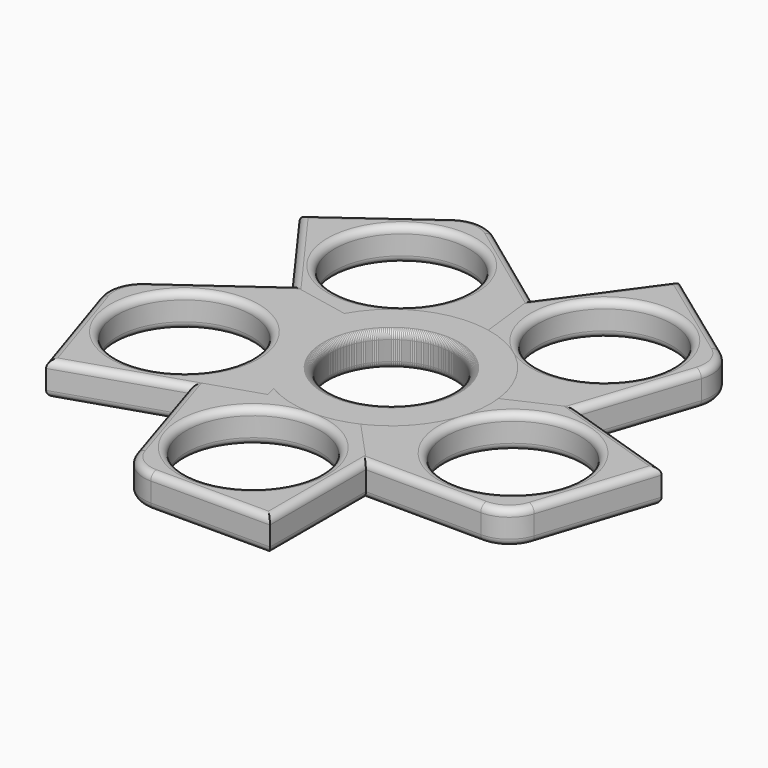
from build123d import *

# Parameters (mm, degrees)
F0_R     = 18.95
F0_R_2   = 10.95
F1_DEPTH = 6
F2_R     = 12.025
F3_DEPTH = 6
F4_R     = 1.27
F5_R     = 1.27
F6_COUNT = 5


# Not quite as in the source:
# - a feature names something its author has since deleted; it is built from what else it names


with BuildPart() as f1:
    # F0 (on Top) → F1 (new body)
    with BuildSketch(Plane.XY):
        Circle(F0_R)
        Circle(F0_R_2, mode=Mode.SUBTRACT)
    extrude(amount=F1_DEPTH)

    # F2 (on face) → F3 (join)
    with BuildSketch(Plane.XY):
        with BuildLine():
            Line((-13.6868354871, -10.5587351833), (-19.1693589182, -20.3174780285))
            Line((-19.1693589182, -20.3174780285), (-12.3887106686, -41.5793495695))
            ThreePointArc((-12.3887106686, -41.5793495695), (-10.0853151337, -44.7770785915), (-6.3389081728, -46))
            Line((-6.3389081728, -46), (15.025, -46))
            Line((15.025, -46), (15.025, -12.1084399137))
            Line((15.025, -12.1084399137), (-13.6868354871, -10.5587351833))
        make_face()
        with Locations((0, -30.975)):
            Circle(F2_R, mode=Mode.SUBTRACT)
    extrude(amount=F3_DEPTH)

    # F4
    f4_edges = [f1.edges().sort_by_distance(p)[0] for p in [
        (-15.779035, -30.948414, 6),
        (15.025, -29.05422, 6),
        (-0.024138, 18.949985, 6),
        (-16.867347, -16.219959, 6),
        (-10.085315, -44.777079, 6),
        (4.343046, -46, 6),
        (14.810585, -12.096867, 6),
        (-10.95, 0, 6),
        (-12.025, -30.975, 6),
    ]]
    fillet(f4_edges, radius=F4_R)

    # F5
    f5_edges = [f1.edges().sort_by_distance(p)[0] for p in [
        (-0.024138, 18.949985, 0),
        (-16.867347, -16.219959, 0),
        (-15.779035, -30.948414, 0),
        (-10.085315, -44.777079, 0),
        (4.343046, -46, 0),
        (15.025, -29.05422, 0),
        (14.810585, -12.096867, 0),
        (-10.95, 0, 0),
        (-12.025, -30.975, 0),
    ]]
    fillet(f5_edges, radius=F5_R)


with BuildPart() as f6_1:
    # F6: instance of F1
    add(f1.part.rotate(Axis((0, 0, 0), (0, 0, 1)), 1 * 360 / F6_COUNT))


with BuildPart() as f6_2:
    # F6: instance of F1
    add(f1.part.rotate(Axis((0, 0, 0), (0, 0, 1)), 2 * 360 / F6_COUNT))


with BuildPart() as f6_3:
    # F6: instance of F1
    add(f1.part.rotate(Axis((0, 0, 0), (0, 0, 1)), 3 * 360 / F6_COUNT))


with BuildPart() as f6_4:
    # F6: instance of F1
    add(f1.part.rotate(Axis((0, 0, 0), (0, 0, 1)), 4 * 360 / F6_COUNT))


solid = Compound([f1.part, f6_1.part, f6_2.part, f6_3.part, f6_4.part])
